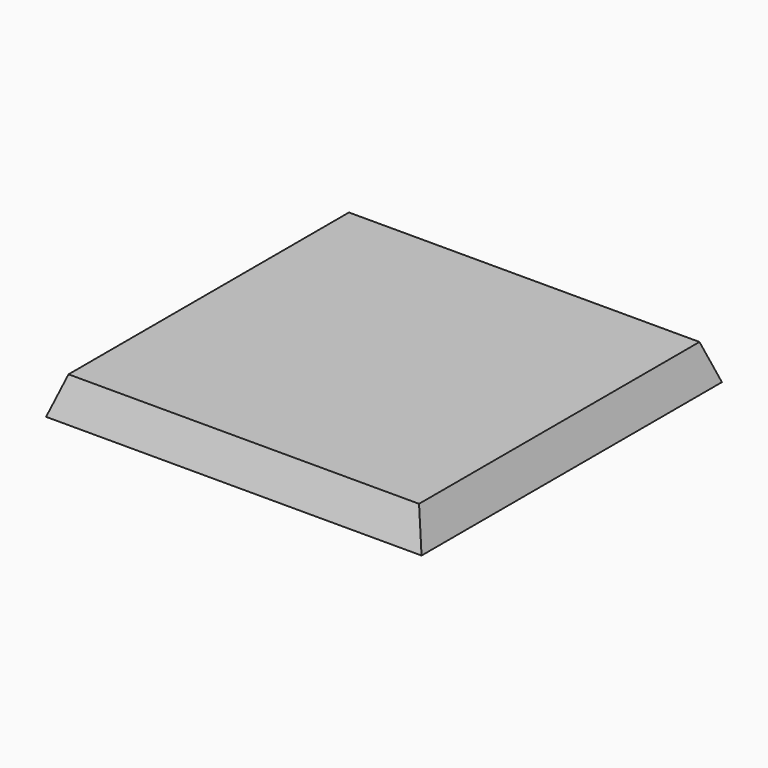
from build123d import *

# Parameters (mm, degrees)
F0_W     = 103.053610972
F0_H     = 103.053610972
F1_DEPTH = 10
F2_SIZE2 = 3.42161
F2_SIZE  = 9.99999
F3_SIZE2 = 3.42161
F3_SIZE  = 9.99999
F4_SIZE2 = 3.42161
F4_SIZE  = 9.99999
F5_SIZE2 = 3.42161
F5_SIZE  = 9.99999


# Not quite as in the source:
# - a fillet or chamfer is up to 0.001 mm smaller than in the source, because OpenCascade refuses the exact size


with BuildPart() as f1:
    # F0 (on Top) → F1 (new body)
    with BuildSketch(Plane.XY):
        with Locations((-4.9147187663, 3.5890949971)):
            Rectangle(F0_W, F0_H)
    extrude(amount=F1_DEPTH)

    # F2 (size 10 and 3.421620486 in the source; OpenCascade refuses exactly that, so slightly less here)
    f2_edges = [f1.edges().sort_by_distance(p)[0] for p in [
        (46.612087, 3.589095, 10),
    ]]
    f2_side = f1.faces().sort_by_distance((46.612087, 3.589095, 5))[0]
    chamfer(f2_edges, length=F2_SIZE, length2=F2_SIZE2, reference=f2_side)

    # F3 (size 10 and 3.421620486 in the source; OpenCascade refuses exactly that, so slightly less here)
    f3_edges = [f1.edges().sort_by_distance(p)[0] for p in [
        (-6.625524, 55.1159, 10),
    ]]
    f3_side = f1.faces().sort_by_distance((-5.765307, 55.1159, 4.971864))[0]
    chamfer(f3_edges, length=F3_SIZE, length2=F3_SIZE2, reference=f3_side)

    # F4 (size 10 and 3.421620486 in the source; OpenCascade refuses exactly that, so slightly less here)
    f4_edges = [f1.edges().sort_by_distance(p)[0] for p in [
        (-6.625524, -47.93771, 10),
    ]]
    f4_side = f1.faces().sort_by_distance((-5.765307, -47.93771, 4.971864))[0]
    chamfer(f4_edges, length=F4_SIZE, length2=F4_SIZE2, reference=f4_side)

    # F5 (size 10 and 3.421620486 in the source; OpenCascade refuses exactly that, so slightly less here)
    f5_edges = [f1.edges().sort_by_distance(p)[0] for p in [
        (-56.441524, 3.589095, 10),
    ]]
    f5_side = f1.faces().sort_by_distance((-56.441524, 3.589095, 4.942762))[0]
    chamfer(f5_edges, length=F5_SIZE, length2=F5_SIZE2, reference=f5_side)


solid = f1.part
